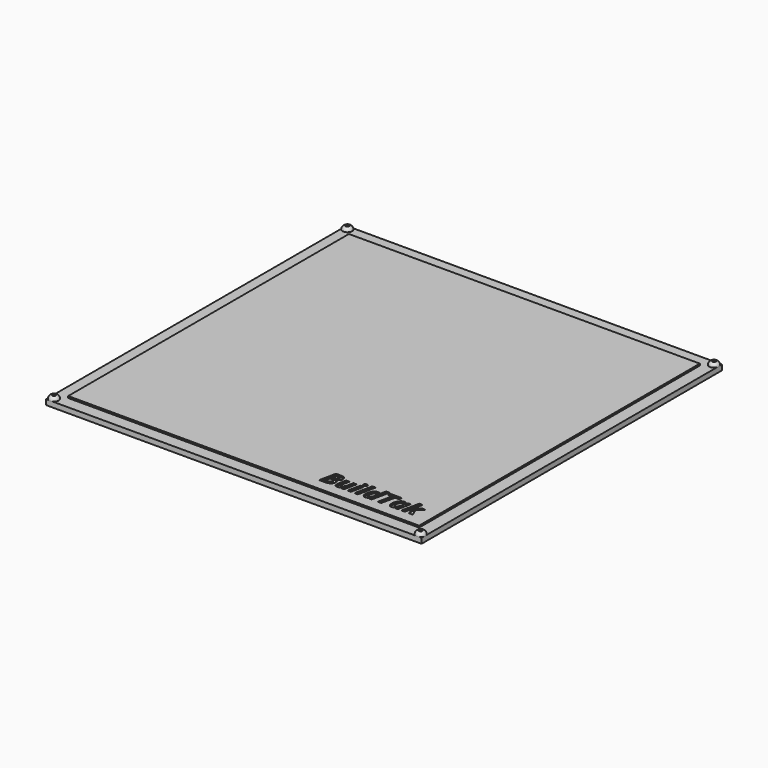
from build123d import *

# Parameters (mm, degrees)
F0_W         = 214
F0_H         = 214
F0_R         = 1.5
F1_DEPTH     = 3
F2_W         = 200
F2_H         = 200
F3_DEPTH     = 1
F4_TEXT_SIZE = 13.2725993408
F5_DEPTH     = 1
F6_R         = 2.75
F6_R_2       = 1.5
F7_DEPTH     = 2
F12_DEPTH    = 1
F14_DEPTH    = 3.5
F15_R        = 2
F16_DEPTH    = 25


# Not quite as in the source:
# - a fillet or chamfer that OpenCascade refuses, or shapes differently, is made with other operations: its cross-section is extruded or revolved along the edge and cut away or added
# - Text() gives the source's letters only with a copy of the font that has no kerning and outlines rounded to 1/6400 em; it was checked with that copy


with BuildPart() as f1:
    # F0 (on Top) → F1 (new body)
    with BuildSketch(Plane.XY):
        Rectangle(F0_W, F0_H)
        with Locations((-104.5, -104.5)):
            Circle(F0_R, mode=Mode.SUBTRACT)
        with Locations((104.5, -104.5)):
            Circle(F0_R, mode=Mode.SUBTRACT)
        with Locations((-104.5, 104.5)):
            Circle(F0_R, mode=Mode.SUBTRACT)
        with Locations((104.5, 104.5)):
            Circle(F0_R, mode=Mode.SUBTRACT)
    extrude(amount=F1_DEPTH)

    # F2 (on face) → F3 (join)
    with BuildSketch(Plane.XY.offset(3)):
        Rectangle(F2_W, F2_H)
    extrude(amount=F3_DEPTH)

    # F4 (on face) → F5 (cut)
    with BuildSketch(Plane.XY.offset(4)):
        with Locations((37.5, -93.5)):
            Text('BuildTak', F4_TEXT_SIZE, font='Open Sans', font_style=FontStyle.BOLDITALIC, text_align=(TextAlign.LEFT, TextAlign.BOTTOM))
    extrude(amount=-F5_DEPTH, mode=Mode.SUBTRACT)

    # F6 (on face) → F7 (join)
    with BuildSketch(Plane.XY.offset(3)):
        with Locations((-104.5, 104.5)):
            Circle(F6_R)
        with Locations((-104.5, 104.5)):
            Circle(F6_R_2, mode=Mode.SUBTRACT)
        with Locations((104.5, 104.5)):
            Circle(F6_R)
        with Locations((104.5, -104.5)):
            Circle(F6_R)
        with Locations((-104.5, -104.5)):
            Circle(F6_R)
        with Locations((-104.5, 104.5)):
            Circle(F6_R_2)
    extrude(amount=F7_DEPTH)

    # F11 (on face) + F10 (on face) + F9 (on face) + F8 (on face) → F12 (cut)
    with BuildSketch(Plane.XY.offset(5)):
        Polygon((104.4976635068, -105.6546981745), (105.4988297062, -105.0793725497), (105.5011661994, -103.9246743752), (104.5023364932, -103.3453018255), (103.5011702938, -103.9206274503), (103.4988338006, -105.0753256248), align=None)
    with BuildSketch(Plane.XY.offset(5)):
        Polygon((-104.4457686749, -105.6534263291), (-103.473987835, -105.0297474593), (-103.5282191601, -103.8763211302), (-104.5542313251, -103.3465736709), (-105.526012165, -103.9702525407), (-105.4717808399, -105.1236788698), align=None)
    with BuildSketch(Plane.XY.offset(5)):
        Polygon((104.5132052756, 103.3453749725), (105.5065372434, 103.9341235904), (105.4933319678, 105.0887486179), (104.4867947244, 105.6546250275), (103.4934627566, 105.0658764096), (103.5066680322, 103.9112513821), align=None)
    with BuildSketch(Plane.XY.offset(5)):
        Polygon((-104.4722507715, 103.3456329381), (-103.4864141849, 103.9468480058), (-103.5141634133, 105.1012150677), (-104.5277492285, 105.6543670619), (-105.5135858151, 105.0531519942), (-105.4858365867, 103.8987849323), align=None)
    extrude(amount=-F12_DEPTH, mode=Mode.SUBTRACT)

    # F13: fillet of radius 2 on 4 edges, made by hand

    # F13_s1 → F13_t2 (revolve, cut)
    with BuildSketch(Plane.XZ.offset(-104.5)):
        with BuildLine():
            ThreePointArc((-101.75, 3), (-102.3357864376, 4.4142135624), (-103.75, 5))
            Line((-103.75, 5), (-101.75, 5))
            Line((-101.75, 5), (-101.75, 3))
        make_face()
    revolve(axis=Axis((-104.5, 104.5, 5), (0, 0, 1)), mode=Mode.SUBTRACT)

    # F13_s3 → F13_t4 (revolve, cut)
    with BuildSketch(Plane.XZ.offset(-104.5)):
        with BuildLine():
            ThreePointArc((107.25, 3), (106.6642135624, 4.4142135624), (105.25, 5))
            Line((105.25, 5), (107.25, 5))
            Line((107.25, 5), (107.25, 3))
        make_face()
    revolve(axis=Axis((104.5, 104.5, 5), (0, 0, 1)), mode=Mode.SUBTRACT)

    # F13_s5 → F13_t6 (revolve, cut)
    with BuildSketch(Plane.XZ.offset(104.5)):
        with BuildLine():
            ThreePointArc((107.25, 3), (106.6642135624, 4.4142135624), (105.25, 5))
            Line((105.25, 5), (107.25, 5))
            Line((107.25, 5), (107.25, 3))
        make_face()
    revolve(axis=Axis((104.5, -104.5, 5), (0, 0, 1)), mode=Mode.SUBTRACT)

    # F13_s7 → F13_t8 (revolve, cut)
    with BuildSketch(Plane.XZ.offset(104.5)):
        with BuildLine():
            ThreePointArc((-101.75, 3), (-102.3357864376, 4.4142135624), (-103.75, 5))
            Line((-103.75, 5), (-101.75, 5))
            Line((-101.75, 5), (-101.75, 3))
        make_face()
    revolve(axis=Axis((-104.5, -104.5, 5), (0, 0, 1)), mode=Mode.SUBTRACT)

    # F14 (add): faces of the model
    f14_faces = [f1.faces().sort_by_distance(p)[0] for p in [
        (-104.5, -104.5, 3),
        (104.5, -104.5, 3),
        (104.5, 104.5, 3),
        (-104.5, 104.5, 3),
    ]]
    extrude(f14_faces, amount=F14_DEPTH)


with BuildPart() as f16:
    # F15 (on Top) → F16 (new body)
    with BuildSketch(Plane.XY):
        Circle(F15_R)
    extrude(amount=F16_DEPTH)


solid = f1.part
